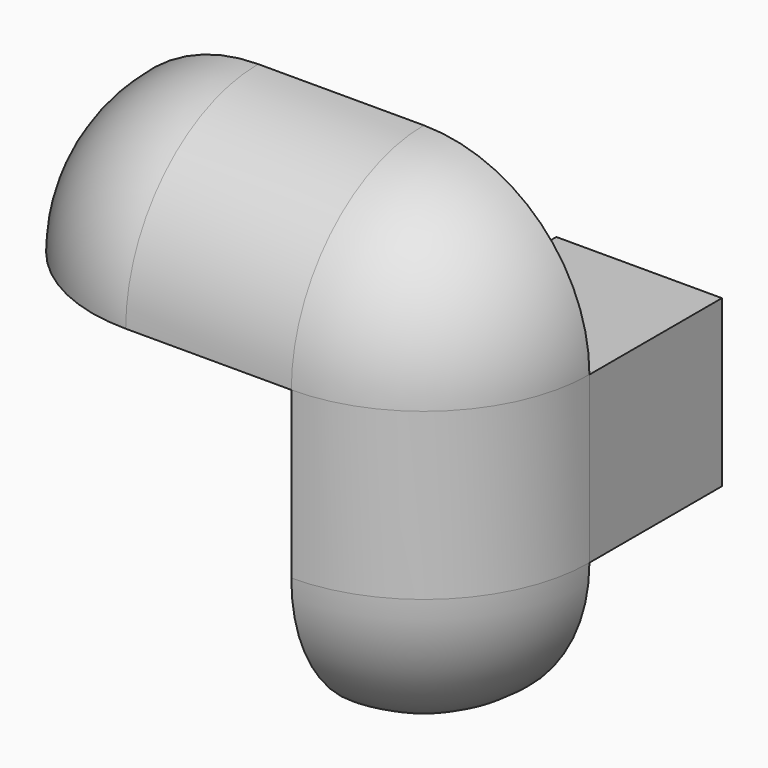
from build123d import *

# Parameters (mm, degrees)
F0_W     = 25.4
F0_H     = 25.4
F1_DEPTH = 76.2
F2_W     = 25.4
F2_H     = 25.4
F3_DEPTH = 50.8
F4_W     = 25.4
F4_H     = 25.4
F5_DEPTH = 25.4
F6_R     = 25.39999


# Not quite as in the source:
# - a fillet or chamfer is up to 0.001 mm smaller than in the source, because OpenCascade refuses the exact size


with BuildPart() as f1:
    # F0 (on Top) → F1 (new body)
    with BuildSketch(Plane.XY):
        with Locations((12.7, 12.7)):
            Rectangle(F0_W, F0_H)
    extrude(amount=F1_DEPTH)

    # F2 (on face) → F3 (join)
    with BuildSketch(Plane(origin=(0, 0, 0), x_dir=(0, -1, 0), z_dir=(-1, 0, 0))):
        with Locations((-12.7, 63.5)):
            Rectangle(F2_W, F2_H)
    extrude(amount=F3_DEPTH)

    # F4 (on face) → F5 (join)
    with BuildSketch(Plane(origin=(0, 25.4, 0), x_dir=(-1, 0, 0), z_dir=(0, 1, 0))):
        with Locations((-12.7, 38.1)):
            Rectangle(F4_W, F4_H)
    extrude(amount=F5_DEPTH)

    # F6 (radius 25.4 in the source; OpenCascade refuses exactly that, so slightly less here)
    f6_edges = [f1.edges().sort_by_distance(p)[0] for p in [
        (-50.8, 12.7, 76.2),
        (-50.8, 0, 63.5),
        (-12.7, 0, 76.2),
        (25.4, 0, 38.1),
        (25.4, 12.7, 0),
        (12.7, 0, 0),
        (25.4, 12.7, 76.2),
    ]]
    fillet(f6_edges, radius=F6_R)


solid = f1.part
